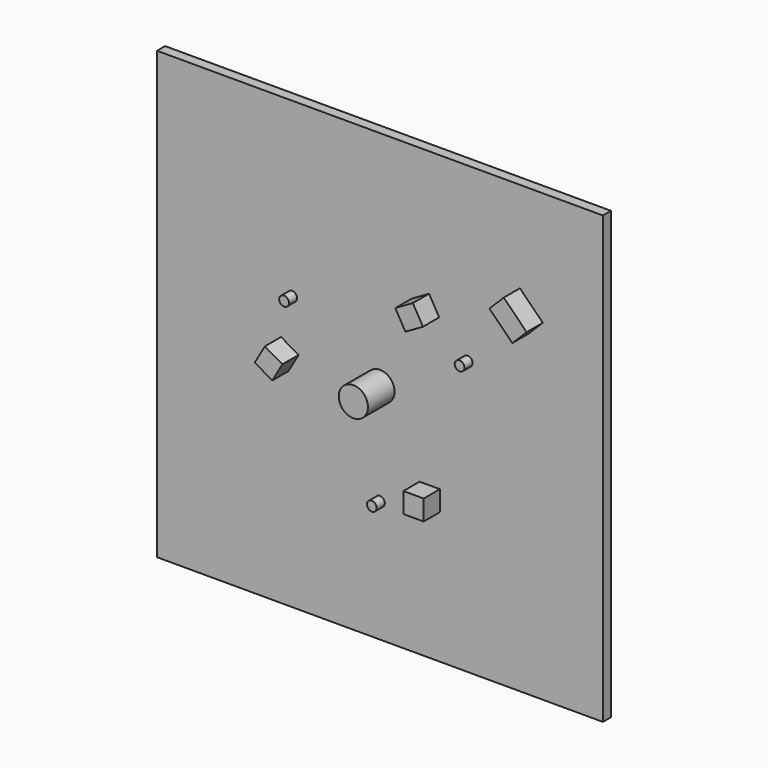
from build123d import *

# Parameters (mm, degrees)
F0_W      = 1100
F0_H      = 1100
F1_DEPTH  = 25
F2_R      = 36.0100678946
F3_DEPTH  = 82
F4_R      = 12
F5_DEPTH  = 25
F6_DEPTH  = 25
F7_W      = 50
F7_H      = 50
F8_DEPTH  = 50
F10_DEPTH = 50


# Not quite as in the source:
# - a feature names something its author has since deleted; it is built from what else it names


with BuildPart() as f1:
    # F0 (on Front) → F1 (new body)
    with BuildSketch(Plane.XZ):
        Rectangle(F0_W, F0_H)
    extrude(amount=F1_DEPTH)

    # F2 (on face) → F3 (join)
    with BuildSketch(Plane.XZ.offset(25)):
        Circle(F2_R)
    extrude(amount=F3_DEPTH)

    # F4 (on face) → F5 (join)
    with BuildSketch(Plane.XZ.offset(25)):
        with Locations((0, -250)):
            Circle(F4_R)
    extrude(amount=F5_DEPTH)

    # F4 (on face) → F6 (join)
    with BuildSketch(Plane.XZ.offset(25)):
        with Locations((-216.5063509461, 125)):
            Circle(F4_R)
        with Locations((216.5063509461, 125)):
            Circle(F4_R)
    extrude(amount=F6_DEPTH)

    # F7 (on face) → F8 (join)
    with BuildSketch(Plane.XZ.offset(25)):
        Polygon((121.1628514659, 240.6145112228), (77.8615812767, 215.6145112228), (102.8615812767, 172.3132410336), (146.1628514659, 197.3132410336), align=None)
        with Locations((122.7968535052, -200.2373629758)):
            Rectangle(F7_W, F7_H)
        Polygon((-268.9597049711, -15.377148247), (-225.6584347818, -40.377148247), (-200.6584347818, 2.9241219422), (-243.9597049711, 27.9241219422), align=None)
    extrude(amount=F8_DEPTH)

    # F9 (on face) → F10 (join)
    with BuildSketch(Plane.XZ.offset(25)):
        Polygon((345.3553390593, 325.3553390593), (310, 290), (366.5685424949, 233.4314575051), (401.9238815543, 268.7867965644), align=None)
    extrude(amount=F10_DEPTH)


solid = f1.part
